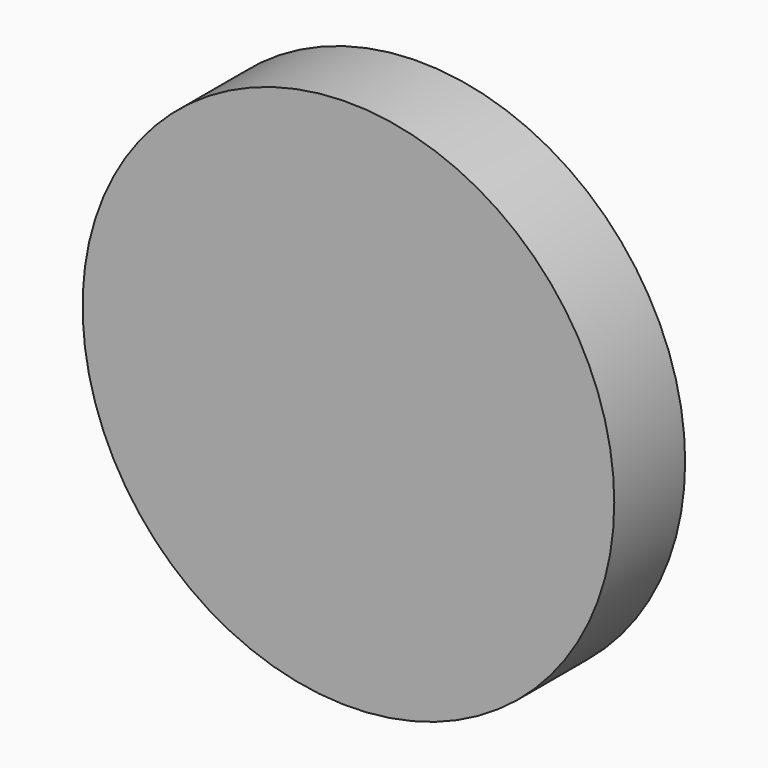
from build123d import *

# Parameters (mm, degrees)
F0_R     = 9
F0_R_2   = 7
F1_DEPTH = 3


# Not quite as in the source:
# - the program builds the solid bodies; features that only make, move or delete a surface that nothing else refers to are left out


with BuildPart() as f1:
    # F0 (on Front) → F1 (new body)
    with BuildSketch(Plane.XZ):
        Circle(F0_R)
        Circle(F0_R_2, mode=Mode.SUBTRACT)
        Circle(F0_R_2)
    extrude(amount=F1_DEPTH)


solid = f1.part
